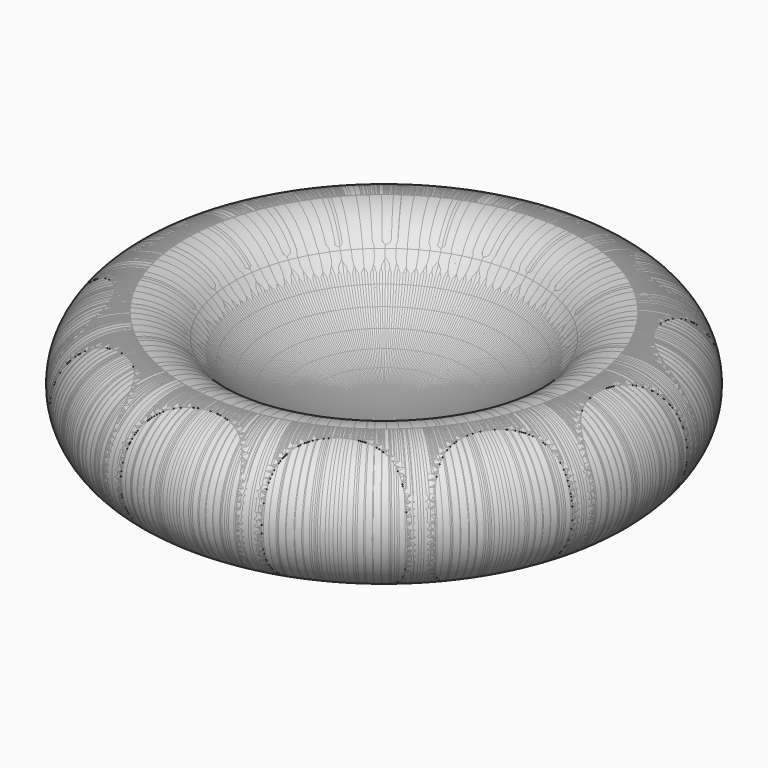
from build123d import *

# Parameters (mm, degrees)
F2_R     = 5.8483090854
F3_DEPTH = 20.574
F4_COUNT = 12


# Not quite as in the source:
# - a feature names something its author has since deleted; it is built from what else it names


with BuildPart() as f1:
    # F0 (on Front) → F1 (revolve)
    with BuildSketch(Plane.XZ):
        with BuildLine():
            ThreePointArc((0, 3.2894316595), (-8.2231201529, 5.1196931504), (-14.8936717517, 10.2649145782))
            ThreePointArc((-14.8936717517, 10.2649145782), (-25.3687490086, 8.9126584587), (-19.7012663795, 0))
            Line((-19.7012663795, 0), (0, 0))
            Line((0, 0), (0, 3.2894316595))
        make_face()
    revolve(axis=Axis((0, 0, 1.6447158298), (0, 0, -1)))

    # F2 (on Top) → F3 (cut)
    with BuildSketch(Plane.XY):
        with Locations((-13.4319122881, 23.2647545257)):
            Circle(F2_R)
        with Locations((0, 26.8638245761)):
            Circle(F2_R)
        with Locations((-13.4319122881, -23.2647545257)):
            Circle(F2_R)
        with Locations((-23.2647545257, -13.4319122881)):
            Circle(F2_R)
        with Locations((-26.8638245761, 0)):
            Circle(F2_R)
        with Locations((-23.2647545257, 13.4319122881)):
            Circle(F2_R)
    extrude(amount=F3_DEPTH, mode=Mode.SUBTRACT)


with BuildPart() as f4_1:
    # F4: instance of F1
    add(f1.part.rotate(Axis((0, 0, 10.2649145782), (0, 0, -1)), 1 * 360 / F4_COUNT))


with BuildPart() as f4_2:
    # F4: instance of F1
    add(f1.part.rotate(Axis((0, 0, 10.2649145782), (0, 0, -1)), 2 * 360 / F4_COUNT))


with BuildPart() as f4_3:
    # F4: instance of F1
    add(f1.part.rotate(Axis((0, 0, 10.2649145782), (0, 0, -1)), 3 * 360 / F4_COUNT))


with BuildPart() as f4_4:
    # F4: instance of F1
    add(f1.part.rotate(Axis((0, 0, 10.2649145782), (0, 0, -1)), 4 * 360 / F4_COUNT))


with BuildPart() as f4_5:
    # F4: instance of F1
    add(f1.part.rotate(Axis((0, 0, 10.2649145782), (0, 0, -1)), 5 * 360 / F4_COUNT))


with BuildPart() as f4_6:
    # F4: instance of F1
    add(f1.part.rotate(Axis((0, 0, 10.2649145782), (0, 0, -1)), 6 * 360 / F4_COUNT))


with BuildPart() as f4_7:
    # F4: instance of F1
    add(f1.part.rotate(Axis((0, 0, 10.2649145782), (0, 0, -1)), 7 * 360 / F4_COUNT))


with BuildPart() as f4_8:
    # F4: instance of F1
    add(f1.part.rotate(Axis((0, 0, 10.2649145782), (0, 0, -1)), 8 * 360 / F4_COUNT))


with BuildPart() as f4_9:
    # F4: instance of F1
    add(f1.part.rotate(Axis((0, 0, 10.2649145782), (0, 0, -1)), 9 * 360 / F4_COUNT))


with BuildPart() as f4_10:
    # F4: instance of F1
    add(f1.part.rotate(Axis((0, 0, 10.2649145782), (0, 0, -1)), 10 * 360 / F4_COUNT))


with BuildPart() as f4_11:
    # F4: instance of F1
    add(f1.part.rotate(Axis((0, 0, 10.2649145782), (0, 0, -1)), 11 * 360 / F4_COUNT))


solid = Compound([f1.part, f4_1.part, f4_2.part, f4_3.part, f4_4.part, f4_5.part, f4_6.part, f4_7.part, f4_8.part, f4_9.part, f4_10.part, f4_11.part])
